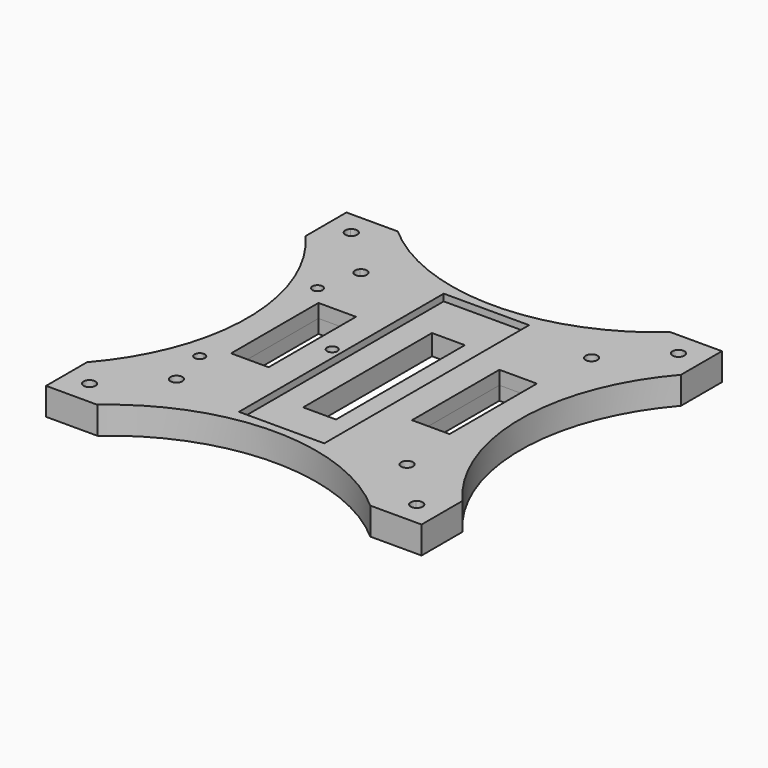
from build123d import *

# Parameters (mm, degrees)
F1_DEPTH = 4
F2_DEPTH = 2
F3_DEPTH = 4


# Not quite as in the source:
# - a feature names something its author has since deleted; it is built from what else it names


with BuildPart() as f1:
    # F0 (on Top) → F1 (new body, symmetric)
    with BuildSketch(Plane.XY):
        with BuildLine():
            Line((55, 40), (55, 55))
            Line((55, 55), (40, 55))
            ThreePointArc((40, 55), (21.3600093633, 43.8733083646), (0, 40))
            Line((0, 40), (0, 37.5))
            Line((0, 37.5), (12.5, 37.5))
            Line((12.5, 37.5), (12.5, 0))
            Line((12.5, 0), (21, 0))
            Line((21, 0), (21, 16))
            Line((21, 16), (32, 16))
            Line((32, 16), (32, 0))
            Line((32, 0), (40, 0))
            ThreePointArc((40, 0), (43.8733083645, 21.3600093633), (55, 40))
        make_face()
        with BuildLine():
            ThreePointArc((35.5367965644, 33.7867965644), (32.1700073825, 33.1171005578), (35.0242334315, 35.0242334315))
            ThreePointArc((35.0242334315, 35.0242334315), (35.4035857463, 34.456492571), (35.5367965644, 33.7867965644))
        make_face(mode=Mode.SUBTRACT)
        with BuildLine():
            ThreePointArc((46.6914953211, 46.6914953211), (46.6914953211, 49.1663690552), (49.1663690552, 49.1663690552))
            ThreePointArc((49.1663690552, 49.1663690552), (49.54572137, 48.5986281948), (49.6789321881, 47.9289321881))
            ThreePointArc((49.6789321881, 47.9289321881), (48.5986281948, 46.3121430062), (46.6914953211, 46.6914953211))
        make_face(mode=Mode.SUBTRACT)
        with BuildLine():
            Line((-12.5, -37.5), (-12.5, 0))
            Line((-12.5, 0), (-13.6673537509, 0))
            ThreePointArc((-13.6673537509, 0), (-15.1673537509, -1.5), (-16.6673537509, 0))
            Line((-16.6673537509, 0), (-21, 0))
            Line((-21, 0), (-21, -16))
            Line((-21, -16), (-32, -16))
            Line((-32, -16), (-32, 0))
            Line((-32, 0), (-36.7343537509, 0))
            Line((-36.7343537509, 0), (-40, 0))
            ThreePointArc((-40, 0), (-43.8733083645, -21.3600093633), (-55, -40))
            Line((-55, -40), (-55, -55))
            Line((-55, -55), (-40, -55))
            ThreePointArc((-40, -55), (-21.3600093633, -43.8733083646), (0, -40))
            Line((0, -40), (0, -37.5))
            Line((0, -37.5), (-12.5, -37.5))
        make_face()
        with BuildLine():
            ThreePointArc((-46.1789321881, -47.9289321881), (-47.2592361815, -49.54572137), (-49.1663690552, -49.1663690552))
            ThreePointArc((-49.1663690552, -49.1663690552), (-49.1663690552, -46.6914953211), (-46.6914953211, -46.6914953211))
            ThreePointArc((-46.6914953211, -46.6914953211), (-46.3121430062, -47.2592361815), (-46.1789321881, -47.9289321881))
        make_face(mode=Mode.SUBTRACT)
        with BuildLine():
            ThreePointArc((-32.0367965644, -33.7867965644), (-33.1171005578, -35.4035857463), (-35.0242334315, -35.0242334315))
            ThreePointArc((-35.0242334315, -35.0242334315), (-34.456492571, -32.1700073825), (-32.0367965644, -33.7867965644))
        make_face(mode=Mode.SUBTRACT)
        with BuildLine():
            ThreePointArc((-35.2343537509, -21.567), (-37.7950139227, -22.6276601718), (-36.7343537509, -20.067))
            ThreePointArc((-36.7343537509, -20.067), (-35.6736935792, -20.5063398282), (-35.2343537509, -21.567))
        make_face(mode=Mode.SUBTRACT)
        with BuildLine():
            Line((0, 37.5), (0, 40))
            ThreePointArc((0, 40), (-21.3600093633, 43.8733083645), (-40, 55))
            Line((-40, 55), (-55, 55))
            Line((-55, 55), (-55, 40))
            ThreePointArc((-55, 40), (-43.8733083646, 21.3600093633), (-40, 0))
            Line((-40, 0), (-36.7343537509, 0))
            Line((-36.7343537509, 0), (-32, 0))
            Line((-32, 0), (-32, 16))
            Line((-32, 16), (-21, 16))
            Line((-21, 16), (-21, 0))
            Line((-21, 0), (-16.6673537509, 0))
            ThreePointArc((-16.6673537509, 0), (-15.1673537509, 1.5), (-13.6673537509, 0))
            Line((-13.6673537509, 0), (-12.5, 0))
            Line((-12.5, 0), (-12.5, 37.5))
            Line((-12.5, 37.5), (0, 37.5))
        make_face()
        with BuildLine():
            ThreePointArc((-35.2343537509, 21.567), (-35.6736935792, 20.5063398282), (-36.7343537509, 20.067))
            ThreePointArc((-36.7343537509, 20.067), (-37.7950139227, 22.6276601718), (-35.2343537509, 21.567))
        make_face(mode=Mode.SUBTRACT)
        with BuildLine():
            ThreePointArc((-32.0367965644, 33.7867965644), (-34.456492571, 32.1700073825), (-35.0242334315, 35.0242334315))
            ThreePointArc((-35.0242334315, 35.0242334315), (-33.1171005578, 35.4035857463), (-32.0367965644, 33.7867965644))
        make_face(mode=Mode.SUBTRACT)
        with BuildLine():
            ThreePointArc((-46.6914953211, 46.6914953211), (-49.1663690552, 46.6914953211), (-49.1663690552, 49.1663690552))
            ThreePointArc((-49.1663690552, 49.1663690552), (-47.2592361815, 49.54572137), (-46.1789321881, 47.9289321881))
            ThreePointArc((-46.1789321881, 47.9289321881), (-46.3121430062, 47.2592361815), (-46.6914953211, 46.6914953211))
        make_face(mode=Mode.SUBTRACT)
        with BuildLine():
            ThreePointArc((55, -40), (43.8733083646, -21.3600093633), (40, 0))
            Line((40, 0), (32, 0))
            Line((32, 0), (32, -16))
            Line((32, -16), (21, -16))
            Line((21, -16), (21, 0))
            Line((21, 0), (12.5, 0))
            Line((12.5, 0), (12.5, -37.5))
            Line((12.5, -37.5), (0, -37.5))
            Line((0, -37.5), (0, -40))
            ThreePointArc((0, -40), (21.3600093633, -43.8733083645), (40, -55))
            Line((40, -55), (55, -55))
            Line((55, -55), (55, -40))
        make_face()
        with BuildLine():
            ThreePointArc((49.6789321881, -47.9289321881), (49.54572137, -48.5986281948), (49.1663690552, -49.1663690552))
            ThreePointArc((49.1663690552, -49.1663690552), (46.6914953211, -49.1663690552), (46.6914953211, -46.6914953211))
            ThreePointArc((46.6914953211, -46.6914953211), (48.5986281948, -46.3121430062), (49.6789321881, -47.9289321881))
        make_face(mode=Mode.SUBTRACT)
        with BuildLine():
            ThreePointArc((35.5367965644, -33.7867965644), (35.4035857463, -34.456492571), (35.0242334315, -35.0242334315))
            ThreePointArc((35.0242334315, -35.0242334315), (32.1700073825, -33.1171005578), (35.5367965644, -33.7867965644))
        make_face(mode=Mode.SUBTRACT)
    extrude(amount=F1_DEPTH, both=True)

    # F0 (on Top) → F2 (join, symmetric)
    with BuildSketch(Plane.XY):
        Polygon((-4.8118475825, 0), (-12.5, 0), (-12.5, -37.5), (0, -37.5), (0, -23.5897935927), (-4.8118475825, -23.5897935927), align=None)
        Polygon((12.5, -37.5), (12.5, 0), (4.8118475825, 0), (4.8118475825, -23.5897935927), (0, -23.5897935927), (0, -37.5), align=None)
        Polygon((0, 23.5897935927), (0, 37.5), (-12.5, 37.5), (-12.5, 0), (-4.8118475825, 0), (-4.8118475825, 23.5897935927), align=None)
        Polygon((12.5, 37.5), (0, 37.5), (0, 23.5897935927), (4.8118475825, 23.5897935927), (4.8118475825, 0), (12.5, 0), align=None)
    extrude(amount=F2_DEPTH, both=True)

    # F0 (on Top) → F3 (join)
    with BuildSketch(Plane.XY):
        Polygon((-4.8118475825, 0), (-12.5, 0), (-12.5, -37.5), (0, -37.5), (0, -23.5897935927), (-4.8118475825, -23.5897935927), align=None)
        Polygon((12.5, -37.5), (12.5, 0), (4.8118475825, 0), (4.8118475825, -23.5897935927), (0, -23.5897935927), (0, -37.5), align=None)
        Polygon((0, 23.5897935927), (0, 37.5), (-12.5, 37.5), (-12.5, 0), (-4.8118475825, 0), (-4.8118475825, 23.5897935927), align=None)
        Polygon((12.5, 37.5), (0, 37.5), (0, 23.5897935927), (4.8118475825, 23.5897935927), (4.8118475825, 0), (12.5, 0), align=None)
    extrude(amount=-F3_DEPTH)


solid = f1.part
